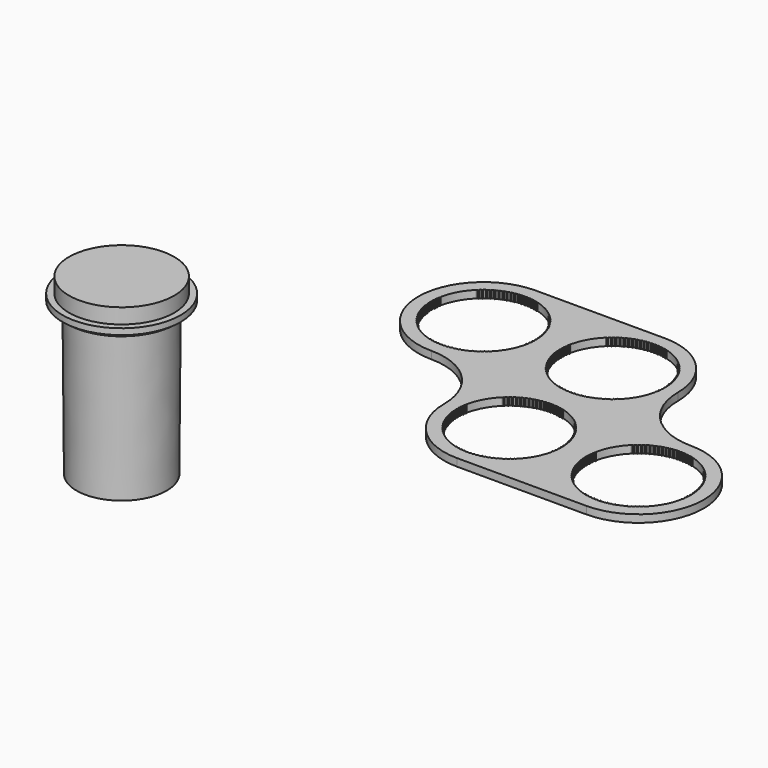
from build123d import *

# Parameters (mm, degrees)
F5_R          = 22.098
F6_DEPTH      = 6.35
F6_DEPTH_BACK = 2.54
F5_R_2        = 24.7948218603
F7_DEPTH      = 2.54
F8_R          = 22.621875
F9_DEPTH      = 1.5875
F10_R         = 19.446875
F12_R         = 18.95078125
F15_DEPTH     = 3.175


# Not quite as in the source:
# - a length typed as a fraction of an inch, garbled in the dataset ("3 / 203.2 mm" for 3/8 in), is restored


with BuildPart() as f6:
    # F5 (on Top) → F6 (new body, two sides)
    with BuildSketch(Plane.XY) as f6_sk:
        Circle(F5_R)
    extrude(amount=F6_DEPTH)
    extrude(f6_sk.sketch, amount=-F6_DEPTH_BACK)

    # F5 (on Top) → F7 (join)
    with BuildSketch(Plane.XY):
        Circle(F5_R_2)
        Circle(F5_R, mode=Mode.SUBTRACT)
    extrude(amount=-F7_DEPTH)


with BuildPart() as f9:
    # F8 (on face) → F9 (new body)
    with BuildSketch(Plane(origin=(0, 0, -2.54), x_dir=(1, 0, 0), z_dir=(0, 0, -1))):
        Circle(F8_R)
    extrude(amount=F9_DEPTH)

    # F10 (on face) → F13 section 0
    with BuildSketch(Plane(origin=(0, 0, -4.1275), x_dir=(1, 0, 0), z_dir=(0, 0, -1))):
        Circle(F10_R)
    # F12 (on offset) → F13 section 1
    with BuildSketch(Plane(origin=(0, 0, -66.83375), x_dir=(1, 0, 0), z_dir=(0, 0, -1))):
        Circle(F12_R)
    loft()


with BuildPart() as f15:
    # F14 (on Top) → F15 (new body)
    with BuildSketch(Plane.XY):
        with BuildLine():
            ThreePointArc((135.5022155802, 0), (143.5290254488, -19.3784332474), (162.9074586963, -27.405243116))
            Line((162.9074586963, -27.405243116), (217.2099449284, -27.405243116))
            ThreePointArc((217.2099449284, -27.405243116), (244.6151880444, 0), (217.2099449284, 27.405243116))
            ThreePointArc((217.2099449284, 27.405243116), (198.1907219258, 35.2832632295), (190.3127018123, 54.3024862321))
            ThreePointArc((190.3127018123, 54.3024862321), (182.2858919437, 73.6809194795), (162.9074586963, 81.7077293481))
            Line((162.9074586963, 81.7077293481), (108.6049724642, 81.7077293481))
            ThreePointArc((108.6049724642, 81.7077293481), (81.1997293481, 54.3024862321), (108.6049724642, 26.897243116))
            ThreePointArc((108.6049724642, 26.897243116), (127.6241954668, 19.0192230026), (135.5022155802, 0))
        make_face()
        with BuildLine():
            Line((184.4449966739, -4.3427294255), (184.3493258728, -4.7928251567))
            ThreePointArc((184.3493258728, -4.7928251567), (182.1607927635, -10.5846099737), (178.4433017857, -15.5358430895))
            Line((178.4433017857, -15.5358430894), (178.1145363694, -15.8577939715))
            Line((178.1145363694, -15.8577939715), (177.6740247135, -15.7247956614))
            Line((177.6740247135, -15.7247956614), (177.7791006262, -16.1727891011))
            Line((177.7791006262, -16.1727891011), (177.4371416893, -16.4806903109))
            Line((177.4371416893, -16.4806903109), (177.0888095533, -16.7813625451))
            Line((177.0888095533, -16.7813625451), (176.6575181795, -16.620966721))
            Line((176.6575181795, -16.620966721), (176.734257008, -17.0746739192))
            Line((176.734257008, -17.0746739192), (176.3736395721, -17.3604957769))
            Line((176.3736395721, -17.3604957769), (176.0071154241, -17.6387027474))
            Line((176.0071154241, -17.6387027474), (175.5867464425, -17.4515424184))
            Line((175.5867464425, -17.4515424184), (175.6348453338, -17.9091728))
            Line((175.6348453338, -17.9091728), (175.2569925911, -18.1717872974))
            Line((175.2569925911, -18.1717872974), (174.8737229346, -18.4264310483))
            Line((174.8737229346, -18.4264310483), (174.4659353494, -18.2132448507))
            Line((174.4659353494, -18.2132448507), (174.4852044791, -18.6729923576))
            Line((174.4852044791, -18.6729923576), (174.0916076417, -18.9113630753))
            Line((174.0916076417, -18.9113630753), (173.6931050669, -19.1414386441))
            Line((173.6931050669, -19.1414386441), (173.2995082295, -18.9030679264))
            Line((173.2995082295, -18.9030679264), (173.2898715512, -19.3631181453))
            Line((173.2898715512, -19.3631181453), (172.882083966, -19.5763043429))
            Line((172.882083966, -19.5763043429), (172.4699211806, -19.7809037265))
            Line((172.4699211806, -19.7809037265), (172.0920684378, -19.518289229))
            Line((172.0920684378, -19.518289229), (172.053563983, -19.9768265519))
            Line((172.053563983, -19.9768265519), (171.6331950014, -20.1639868809))
            Line((171.6331950014, -20.1639868809), (171.2089986235, -20.3423026189))
            Line((171.2089986235, -20.3423026189), (170.8483811875, -20.0564807611))
            Line((170.8483811875, -20.0564807611), (170.7811609157, -20.5116955506))
            Line((170.7811609157, -20.5116955506), (170.349869542, -20.6720913747))
            Line((170.349869542, -20.6720913747), (169.9153136809, -20.8234197363))
            Line((169.9153136809, -20.8234197363), (169.573354744, -20.5155185266))
            Line((169.573354744, -20.5155185266), (169.4776839429, -20.9656142578))
            Line((169.4776839429, -20.9656142578), (169.0371722871, -21.098612568))
            Line((169.0371722871, -21.098612568), (168.5939719362, -21.2223563294))
            Line((168.5939719362, -21.2223563294), (168.2720210541, -20.8935909131))
            Line((168.2720210541, -20.8935909131), (168.1482772927, -21.3367912639))
            Line((168.1482772927, -21.3367912639), (167.700283853, -21.4418671766))
            Line((167.700283853, -21.4418671766), (167.2501881217, -21.5375379776))
            Line((167.2501881217, -21.5375379776), (166.9495158875, -21.1892058416))
            Line((166.9495158875, -21.1892058416), (166.7981875258, -21.6237617027))
            Line((166.7981875258, -21.6237617027), (166.3444803277, -21.7005005312))
            Line((166.3444803277, -21.7005005312), (165.8892655382, -21.767720803))
            Line((165.8892655382, -21.767720803), (165.6110585677, -21.4011966551))
            Line((165.6110585677, -21.4011966551), (165.4327428297, -21.825393033))
            Line((165.4327428297, -21.825393033), (164.9751124482, -21.8734919243))
            Line((164.9751124482, -21.8734919243), (164.5165751254, -21.9119963791))
            Line((164.5165751254, -21.9119963791), (164.2619313744, -21.5287267226))
            Line((164.2619313744, -21.5287267226), (164.0573319909, -21.9408895081))
            Line((164.0573319909, -21.9408895081), (163.597584484, -21.9601586378))
            Line((163.597584484, -21.9601586378), (163.1375342651, -21.9697953161))
            Line((163.1375342651, -21.9697953161), (162.9074586963, -21.5712927414))
            Line((162.9074586963, -21.5712927414), (162.6773831275, -21.9697953161))
            Line((162.6773831275, -21.9697953161), (162.2173329086, -21.9601586378))
            Line((162.2173329086, -21.9601586378), (161.7575854017, -21.9408895081))
            Line((161.7575854017, -21.9408895081), (161.5529860181, -21.5287267226))
            Line((161.5529860181, -21.5287267226), (161.2983422672, -21.9119963791))
            Line((161.2983422672, -21.9119963791), (160.8398049443, -21.8734919243))
            Line((160.8398049443, -21.8734919243), (160.3821745628, -21.825393033))
            Line((160.3821745628, -21.825393033), (160.2038588248, -21.4011966551))
            Line((160.2038588248, -21.4011966551), (159.9256518543, -21.767720803))
            Line((159.9256518543, -21.767720803), (159.4704370649, -21.7005005312))
            Line((159.4704370649, -21.7005005312), (159.0167298667, -21.6237617027))
            Line((159.0167298667, -21.6237617027), (158.8654015051, -21.1892058416))
            Line((158.8654015051, -21.1892058416), (158.5647292708, -21.5375379776))
            Line((158.5647292708, -21.5375379776), (158.1146335395, -21.4418671766))
            Line((158.1146335395, -21.4418671766), (157.6666400998, -21.3367912639))
            Line((157.6666400998, -21.3367912639), (157.5428963384, -20.8935909131))
            Line((157.5428963384, -20.8935909131), (157.2209454563, -21.2223563294))
            Line((157.2209454563, -21.2223563294), (156.7777451055, -21.098612568))
            ThreePointArc((156.7777451055, -21.098612568), (152.3228487226, -19.2533340672), (148.3777757032, -16.4806903108))
            Line((148.3777757032, -16.4806903109), (148.0358167664, -16.1727891011))
            Line((148.0358167664, -16.1727891011), (148.140892679, -15.7247956614))
            Line((148.140892679, -15.7247956614), (147.7003810232, -15.8577939715))
            Line((147.7003810232, -15.8577939715), (147.3716156068, -15.5358430894))
            Line((147.3716156068, -15.5358430894), (147.0496647247, -15.2070776731))
            Line((147.0496647247, -15.2070776731), (147.1826630349, -14.7665660172))
            Line((147.1826630349, -14.7665660172), (146.7346695952, -14.8716419299))
            Line((146.7346695952, -14.8716419299), (146.4267683854, -14.529682993))
            Line((146.4267683854, -14.529682993), (146.1260961511, -14.181350857))
            Line((146.1260961511, -14.181350857), (146.2864919753, -13.7500594832))
            Line((146.2864919753, -13.7500594832), (145.8327847771, -13.8267983118))
            Line((145.8327847771, -13.8267983118), (145.5469629194, -13.4661808758))
            Line((145.5469629194, -13.4661808758), (145.2687559488, -13.0996567279))
            Line((145.2687559488, -13.0996567279), (145.4559162779, -12.6792877463))
            Line((145.4559162779, -12.6792877463), (144.9982858963, -12.7273866375))
            Line((144.9982858963, -12.7273866375), (144.7356713989, -12.3495338948))
            Line((144.7356713989, -12.3495338948), (144.4810276479, -11.9662642383))
            Line((144.4810276479, -11.9662642383), (144.6942138456, -11.5584766532))
            Line((144.6942138456, -11.5584766532), (144.2344663387, -11.5777457829))
            Line((144.2344663387, -11.5777457829), (143.996095621, -11.1841489455))
            Line((143.996095621, -11.1841489455), (143.7660200521, -10.7856463707))
            Line((143.7660200521, -10.7856463707), (144.0043907698, -10.3920495333))
            Line((144.0043907698, -10.3920495333), (143.544340551, -10.3824128549))
            Line((143.544340551, -10.3824128549), (143.3311543533, -9.9746252698))
            Line((143.3311543533, -9.9746252698), (143.1265549698, -9.5624624843))
            Line((143.1265549698, -9.5624624843), (143.3891694672, -9.1846097416))
            Line((143.3891694672, -9.1846097416), (142.9306321444, -9.1461052868))
            Line((142.9306321444, -9.1461052868), (142.7434718154, -8.7257363051))
            Line((142.7434718154, -8.7257363051), (142.5651560774, -8.3015399272))
            Line((142.5651560774, -8.3015399272), (142.8509779351, -7.9409224912))
            Line((142.8509779351, -7.9409224912), (142.3957631457, -7.8737022195))
            Line((142.3957631457, -7.8737022195), (142.2353673216, -7.4424108457))
            Line((142.2353673216, -7.4424108457), (142.0840389599, -7.0078549846))
            Line((142.0840389599, -7.0078549846), (142.3919401697, -6.6658960477))
            Line((142.3919401697, -6.6658960477), (141.9418444384, -6.5702252467))
            Line((141.9418444384, -6.5702252467), (141.8088461283, -6.1297135908))
            Line((141.8088461283, -6.1297135908), (141.6851023669, -5.6865132399))
            Line((141.6851023669, -5.6865132399), (142.0138677832, -5.3645623578))
            Line((142.0138677832, -5.3645623578), (141.5706674324, -5.2408185965))
            Line((141.5706674324, -5.2408185965), (141.4655915197, -4.7928251567))
            Line((141.4655915197, -4.7928251567), (141.3699207187, -4.3427294255))
            Line((141.3699207187, -4.3427294255), (141.7182528547, -4.0420571912))
            Line((141.7182528547, -4.0420571912), (141.2836969936, -3.8907288296))
            Line((141.2836969936, -3.8907288296), (141.2069581651, -3.4370216314))
            Line((141.2069581651, -3.4370216314), (141.1397378933, -2.981806842))
            Line((141.1397378933, -2.981806842), (141.5062620412, -2.7035998714))
            Line((141.5062620412, -2.7035998714), (141.0820656633, -2.5252841335))
            Line((141.0820656633, -2.5252841335), (141.033966772, -2.0676537519))
            Line((141.033966772, -2.0676537519), (140.9954623172, -1.6091164291))
            Line((140.9954623172, -1.6091164291), (141.3787319736, -1.3544726781))
            Line((141.3787319736, -1.3544726781), (140.9665691882, -1.1498732946))
            Line((140.9665691882, -1.1498732946), (140.9473000585, -0.6901257877))
            Line((140.9473000585, -0.6901257877), (140.9376633801, -0.2300755688))
            Line((140.9376633801, -0.2300755688), (141.3361659549, 0))
            Line((141.3361659549, 0), (140.9376633801, 0.2300755688))
            Line((140.9376633801, 0.2300755688), (140.9473000585, 0.6901257877))
            Line((140.9473000585, 0.6901257877), (140.9665691882, 1.1498732946))
            Line((140.9665691882, 1.1498732946), (141.3787319736, 1.3544726781))
            Line((141.3787319736, 1.3544726781), (140.9954623172, 1.6091164291))
            Line((140.9954623172, 1.6091164291), (141.033966772, 2.0676537519))
            Line((141.033966772, 2.0676537519), (141.0820656633, 2.5252841335))
            Line((141.0820656633, 2.5252841335), (141.5062620412, 2.7035998714))
            Line((141.5062620412, 2.7035998714), (141.1397378933, 2.981806842))
            Line((141.1397378933, 2.981806842), (141.2069581651, 3.4370216314))
            Line((141.2069581651, 3.4370216314), (141.2836969936, 3.8907288296))
            Line((141.2836969936, 3.8907288296), (141.7182528547, 4.0420571912))
            Line((141.7182528547, 4.0420571912), (141.3699207187, 4.3427294255))
            Line((141.3699207187, 4.3427294255), (141.4655915197, 4.7928251567))
            ThreePointArc((141.4655915197, 4.7928251567), (143.654124629, 10.5846099737), (147.3716156068, 15.5358430894))
            Line((147.3716156068, 15.5358430894), (147.7003810232, 15.8577939715))
            Line((147.7003810232, 15.8577939715), (148.140892679, 15.7247956614))
            Line((148.140892679, 15.7247956614), (148.0358167664, 16.1727891011))
            Line((148.0358167664, 16.1727891011), (148.3777757032, 16.4806903109))
            Line((148.3777757032, 16.4806903109), (148.7261078393, 16.7813625451))
            Line((148.7261078393, 16.7813625451), (149.157399213, 16.620966721))
            Line((149.157399213, 16.620966721), (149.0806603845, 17.0746739192))
            Line((149.0806603845, 17.0746739192), (149.4412778205, 17.3604957769))
            Line((149.4412778205, 17.3604957769), (149.8078019684, 17.6387027474))
            Line((149.8078019684, 17.6387027474), (150.22817095, 17.4515424184))
            Line((150.22817095, 17.4515424184), (150.1800720587, 17.9091728))
            Line((150.1800720587, 17.9091728), (150.5579248015, 18.1717872974))
            Line((150.5579248015, 18.1717872974), (150.941194458, 18.4264310483))
            Line((150.941194458, 18.4264310483), (151.3489820431, 18.2132448507))
            Line((151.3489820431, 18.2132448507), (151.3297129134, 18.6729923576))
            Line((151.3297129134, 18.6729923576), (151.7233097508, 18.9113630753))
            Line((151.7233097508, 18.9113630753), (152.1218123256, 19.1414386441))
            Line((152.1218123256, 19.1414386441), (152.515409163, 18.9030679264))
            Line((152.515409163, 18.9030679264), (152.5250458413, 19.3631181453))
            Line((152.5250458413, 19.3631181453), (152.9328334265, 19.5763043429))
            Line((152.9328334265, 19.5763043429), (153.344996212, 19.7809037265))
            Line((153.344996212, 19.7809037265), (153.7228489547, 19.518289229))
            Line((153.7228489547, 19.518289229), (153.7613534095, 19.9768265519))
            Line((153.7613534095, 19.9768265519), (154.1817223911, 20.1639868809))
            Line((154.1817223911, 20.1639868809), (154.6059187691, 20.3423026189))
            Line((154.6059187691, 20.3423026189), (154.966536205, 20.0564807611))
            Line((154.966536205, 20.0564807611), (155.0337564768, 20.5116955506))
            Line((155.0337564768, 20.5116955506), (155.4650478506, 20.6720913747))
            Line((155.4650478506, 20.6720913747), (155.8996037117, 20.8234197363))
            Line((155.8996037117, 20.8234197363), (156.2415626486, 20.5155185266))
            Line((156.2415626486, 20.5155185266), (156.3372334496, 20.9656142578))
            Line((156.3372334496, 20.9656142578), (156.7777451055, 21.098612568))
            Line((156.7777451055, 21.098612568), (157.2209454563, 21.2223563294))
            Line((157.2209454563, 21.2223563294), (157.5428963384, 20.8935909131))
            Line((157.5428963384, 20.8935909131), (157.6666400998, 21.3367912639))
            Line((157.6666400998, 21.3367912639), (158.1146335395, 21.4418671766))
            Line((158.1146335395, 21.4418671766), (158.5647292708, 21.5375379776))
            Line((158.5647292708, 21.5375379776), (158.8654015051, 21.1892058416))
            Line((158.8654015051, 21.1892058416), (159.0167298667, 21.6237617027))
            Line((159.0167298667, 21.6237617027), (159.4704370649, 21.7005005312))
            Line((159.4704370649, 21.7005005312), (159.9256518543, 21.767720803))
            Line((159.9256518543, 21.767720803), (160.2038588248, 21.4011966551))
            Line((160.2038588248, 21.4011966551), (160.3821745628, 21.825393033))
            Line((160.3821745628, 21.825393033), (160.8398049443, 21.8734919243))
            Line((160.8398049443, 21.8734919243), (161.2983422672, 21.9119963791))
            Line((161.2983422672, 21.9119963791), (161.5529860181, 21.5287267226))
            Line((161.5529860181, 21.5287267226), (161.7575854017, 21.9408895081))
            Line((161.7575854017, 21.9408895081), (162.2173329086, 21.9601586378))
            Line((162.2173329086, 21.9601586378), (162.6773831275, 21.9697953161))
            Line((162.6773831275, 21.9697953161), (162.9074586963, 21.5712927414))
            Line((162.9074586963, 21.5712927414), (163.1375342651, 21.9697953161))
            Line((163.1375342651, 21.9697953161), (163.597584484, 21.9601586378))
            Line((163.597584484, 21.9601586378), (164.0573319909, 21.9408895081))
            Line((164.0573319909, 21.9408895081), (164.2619313744, 21.5287267226))
            Line((164.2619313744, 21.5287267226), (164.5165751254, 21.9119963791))
            Line((164.5165751254, 21.9119963791), (164.9751124482, 21.8734919243))
            Line((164.9751124482, 21.8734919243), (165.4327428297, 21.825393033))
            Line((165.4327428297, 21.825393033), (165.6110585677, 21.4011966551))
            Line((165.6110585677, 21.4011966551), (165.8892655382, 21.767720803))
            Line((165.8892655382, 21.767720803), (166.3444803277, 21.7005005312))
            Line((166.3444803277, 21.7005005312), (166.7981875258, 21.6237617027))
            Line((166.7981875258, 21.6237617027), (166.9495158875, 21.1892058416))
            Line((166.9495158875, 21.1892058416), (167.2501881217, 21.5375379776))
            Line((167.2501881217, 21.5375379776), (167.700283853, 21.4418671766))
            Line((167.700283853, 21.4418671766), (168.1482772927, 21.3367912639))
            Line((168.1482772927, 21.3367912639), (168.2720210541, 20.8935909131))
            Line((168.2720210541, 20.8935909131), (168.5939719362, 21.2223563294))
            Line((168.5939719362, 21.2223563294), (169.0371722871, 21.098612568))
            ThreePointArc((169.0371722871, 21.098612568), (173.49206867, 19.2533340672), (177.4371416893, 16.4806903109))
            Line((177.4371416893, 16.4806903109), (177.7791006262, 16.1727891011))
            Line((177.7791006262, 16.1727891011), (177.6740247135, 15.7247956614))
            Line((177.6740247135, 15.7247956614), (178.1145363694, 15.8577939715))
            Line((178.1145363694, 15.8577939715), (178.4433017857, 15.5358430894))
            Line((178.4433017857, 15.5358430894), (178.7652526678, 15.2070776731))
            Line((178.7652526678, 15.2070776731), (178.6322543576, 14.7665660172))
            Line((178.6322543576, 14.7665660172), (179.0802477974, 14.8716419299))
            Line((179.0802477974, 14.8716419299), (179.3881490071, 14.529682993))
            Line((179.3881490071, 14.529682993), (179.6888212414, 14.181350857))
            Line((179.6888212414, 14.181350857), (179.5284254173, 13.7500594832))
            Line((179.5284254173, 13.7500594832), (179.9821326154, 13.8267983118))
            Line((179.9821326154, 13.8267983118), (180.2679544732, 13.4661808758))
            Line((180.2679544732, 13.4661808758), (180.5461614437, 13.0996567279))
            Line((180.5461614437, 13.0996567279), (180.3590011147, 12.6792877463))
            Line((180.3590011147, 12.6792877463), (180.8166314962, 12.7273866375))
            Line((180.8166314962, 12.7273866375), (181.0792459937, 12.3495338948))
            Line((181.0792459937, 12.3495338948), (181.3338897446, 11.9662642383))
            Line((181.3338897446, 11.9662642383), (181.120703547, 11.5584766532))
            Line((181.120703547, 11.5584766532), (181.5804510539, 11.5777457829))
            Line((181.5804510539, 11.5777457829), (181.8188217716, 11.1841489455))
            Line((181.8188217716, 11.1841489455), (182.0488973404, 10.7856463707))
            Line((182.0488973404, 10.7856463707), (181.8105266227, 10.3920495333))
            Line((181.8105266227, 10.3920495333), (182.2705768416, 10.3824128549))
            Line((182.2705768416, 10.3824128549), (182.4837630392, 9.9746252698))
            Line((182.4837630392, 9.9746252698), (182.6883624227, 9.5624624843))
            Line((182.6883624227, 9.5624624843), (182.4257479253, 9.1846097416))
            Line((182.4257479253, 9.1846097416), (182.8842852481, 9.1461052868))
            Line((182.8842852481, 9.1461052868), (183.0714455772, 8.7257363051))
            Line((183.0714455772, 8.7257363051), (183.2497613151, 8.3015399272))
            Line((183.2497613151, 8.3015399272), (182.9639394574, 7.9409224912))
            Line((182.9639394574, 7.9409224912), (183.4191542468, 7.8737022195))
            Line((183.4191542468, 7.8737022195), (183.579550071, 7.4424108457))
            Line((183.579550071, 7.4424108457), (183.7308784326, 7.0078549846))
            Line((183.7308784326, 7.0078549846), (183.4229772228, 6.6658960477))
            Line((183.4229772228, 6.6658960477), (183.8730729541, 6.5702252467))
            Line((183.8730729541, 6.5702252467), (184.0060712643, 6.1297135908))
            Line((184.0060712643, 6.1297135908), (184.1298150257, 5.6865132399))
            Line((184.1298150257, 5.6865132399), (183.8010496093, 5.3645623578))
            Line((183.8010496093, 5.3645623578), (184.2442499602, 5.2408185965))
            Line((184.2442499602, 5.2408185965), (184.3493258728, 4.7928251567))
            Line((184.3493258728, 4.7928251567), (184.4449966739, 4.3427294255))
            Line((184.4449966739, 4.3427294255), (184.0966645378, 4.0420571912))
            Line((184.0966645378, 4.0420571912), (184.531220399, 3.8907288296))
            Line((184.531220399, 3.8907288296), (184.6079592275, 3.4370216314))
            Line((184.6079592275, 3.4370216314), (184.6751794993, 2.981806842))
            Line((184.6751794993, 2.981806842), (184.3086553513, 2.7035998714))
            Line((184.3086553513, 2.7035998714), (184.7328517293, 2.5252841335))
            Line((184.7328517293, 2.5252841335), (184.7809506206, 2.0676537519))
            Line((184.7809506206, 2.0676537519), (184.8194550754, 1.6091164291))
            Line((184.8194550754, 1.6091164291), (184.4361854189, 1.3544726781))
            Line((184.4361854189, 1.3544726781), (184.8483482044, 1.1498732946))
            Line((184.8483482044, 1.1498732946), (184.8676173341, 0.6901257877))
            Line((184.8676173341, 0.6901257877), (184.8772540124, 0.2300755688))
            Line((184.8772540124, 0.2300755688), (184.4787514376, 0))
            Line((184.4787514376, 0), (184.8772540124, -0.2300755688))
            Line((184.8772540124, -0.2300755688), (184.8676173341, -0.6901257877))
            Line((184.8676173341, -0.6901257877), (184.8483482044, -1.1498732946))
            Line((184.8483482044, -1.1498732946), (184.4361854189, -1.3544726781))
            Line((184.4361854189, -1.3544726781), (184.8194550754, -1.6091164291))
            Line((184.8194550754, -1.6091164291), (184.7809506206, -2.0676537519))
            Line((184.7809506206, -2.0676537519), (184.7328517293, -2.5252841335))
            Line((184.7328517293, -2.5252841335), (184.3086553513, -2.7035998714))
            Line((184.3086553513, -2.7035998714), (184.6751794993, -2.981806842))
            Line((184.6751794993, -2.981806842), (184.6079592275, -3.4370216314))
            Line((184.6079592275, -3.4370216314), (184.531220399, -3.8907288296))
            Line((184.531220399, -3.8907288296), (184.0966645378, -4.0420571912))
            Line((184.0966645378, -4.0420571912), (184.4449966739, -4.3427294255))
        make_face(mode=Mode.SUBTRACT)
        with BuildLine():
            Line((238.747482906, -4.3427294255), (238.6518121049, -4.7928251567))
            ThreePointArc((238.6518121049, -4.7928251567), (236.4632789956, -10.5846099737), (232.7457880178, -15.5358430895))
            Line((232.7457880178, -15.5358430894), (232.4170226015, -15.8577939715))
            Line((232.4170226015, -15.8577939715), (231.9765109456, -15.7247956614))
            Line((231.9765109456, -15.7247956614), (232.0815868583, -16.1727891011))
            Line((232.0815868583, -16.1727891011), (231.7396279214, -16.4806903109))
            Line((231.7396279214, -16.4806903109), (231.3912957853, -16.7813625451))
            Line((231.3912957853, -16.7813625451), (230.9600044116, -16.620966721))
            Line((230.9600044116, -16.620966721), (231.0367432401, -17.0746739192))
            Line((231.0367432401, -17.0746739192), (230.6761258042, -17.3604957769))
            Line((230.6761258042, -17.3604957769), (230.3096016562, -17.6387027474))
            Line((230.3096016562, -17.6387027474), (229.8892326746, -17.4515424184))
            Line((229.8892326746, -17.4515424184), (229.9373315659, -17.9091728))
            Line((229.9373315659, -17.9091728), (229.5594788231, -18.1717872974))
            Line((229.5594788231, -18.1717872974), (229.1762091667, -18.4264310483))
            Line((229.1762091667, -18.4264310483), (228.7684215815, -18.2132448507))
            Line((228.7684215815, -18.2132448507), (228.7876907112, -18.6729923576))
            Line((228.7876907112, -18.6729923576), (228.3940938738, -18.9113630753))
            Line((228.3940938738, -18.9113630753), (227.995591299, -19.1414386441))
            Line((227.995591299, -19.1414386441), (227.6019944616, -18.9030679264))
            Line((227.6019944616, -18.9030679264), (227.5923577833, -19.3631181453))
            Line((227.5923577833, -19.3631181453), (227.1845701981, -19.5763043429))
            Line((227.1845701981, -19.5763043429), (226.7724074127, -19.7809037265))
            Line((226.7724074127, -19.7809037265), (226.3945546699, -19.518289229))
            Line((226.3945546699, -19.518289229), (226.3560502151, -19.9768265519))
            Line((226.3560502151, -19.9768265519), (225.9356812335, -20.1639868809))
            Line((225.9356812335, -20.1639868809), (225.5114848555, -20.3423026189))
            Line((225.5114848555, -20.3423026189), (225.1508674196, -20.0564807611))
            Line((225.1508674196, -20.0564807611), (225.0836471478, -20.5116955506))
            Line((225.0836471478, -20.5116955506), (224.6523557741, -20.6720913747))
            Line((224.6523557741, -20.6720913747), (224.2177999129, -20.8234197363))
            Line((224.2177999129, -20.8234197363), (223.8758409761, -20.5155185266))
            Line((223.8758409761, -20.5155185266), (223.780170175, -20.9656142578))
            Line((223.780170175, -20.9656142578), (223.3396585191, -21.098612568))
            Line((223.3396585191, -21.098612568), (222.8964581683, -21.2223563294))
            Line((222.8964581683, -21.2223563294), (222.5745072862, -20.8935909131))
            Line((222.5745072862, -20.8935909131), (222.4507635248, -21.3367912639))
            Line((222.4507635248, -21.3367912639), (222.0027700851, -21.4418671766))
            Line((222.0027700851, -21.4418671766), (221.5526743538, -21.5375379776))
            Line((221.5526743538, -21.5375379776), (221.2520021195, -21.1892058416))
            Line((221.2520021195, -21.1892058416), (221.1006737579, -21.6237617027))
            Line((221.1006737579, -21.6237617027), (220.6469665598, -21.7005005312))
            Line((220.6469665598, -21.7005005312), (220.1917517703, -21.767720803))
            Line((220.1917517703, -21.767720803), (219.9135447998, -21.4011966551))
            Line((219.9135447998, -21.4011966551), (219.7352290618, -21.825393033))
            Line((219.7352290618, -21.825393033), (219.2775986803, -21.8734919243))
            Line((219.2775986803, -21.8734919243), (218.8190613575, -21.9119963791))
            Line((218.8190613575, -21.9119963791), (218.5644176065, -21.5287267226))
            Line((218.5644176065, -21.5287267226), (218.359818223, -21.9408895081))
            Line((218.359818223, -21.9408895081), (217.9000707161, -21.9601586378))
            Line((217.9000707161, -21.9601586378), (217.4400204972, -21.9697953161))
            Line((217.4400204972, -21.9697953161), (217.2099449284, -21.5712927414))
            Line((217.2099449284, -21.5712927414), (216.9798693595, -21.9697953161))
            Line((216.9798693595, -21.9697953161), (216.5198191407, -21.9601586378))
            Line((216.5198191407, -21.9601586378), (216.0600716337, -21.9408895081))
            Line((216.0600716337, -21.9408895081), (215.8554722502, -21.5287267226))
            Line((215.8554722502, -21.5287267226), (215.6008284993, -21.9119963791))
            Line((215.6008284993, -21.9119963791), (215.1422911764, -21.8734919243))
            Line((215.1422911764, -21.8734919243), (214.6846607949, -21.825393033))
            Line((214.6846607949, -21.825393033), (214.5063450569, -21.4011966551))
            Line((214.5063450569, -21.4011966551), (214.2281380864, -21.767720803))
            Line((214.2281380864, -21.767720803), (213.772923297, -21.7005005312))
            Line((213.772923297, -21.7005005312), (213.3192160988, -21.6237617027))
            Line((213.3192160988, -21.6237617027), (213.1678877372, -21.1892058416))
            Line((213.1678877372, -21.1892058416), (212.8672155029, -21.5375379776))
            Line((212.8672155029, -21.5375379776), (212.4171197716, -21.4418671766))
            Line((212.4171197716, -21.4418671766), (211.9691263319, -21.3367912639))
            Line((211.9691263319, -21.3367912639), (211.8453825705, -20.8935909131))
            Line((211.8453825705, -20.8935909131), (211.5234316884, -21.2223563294))
            Line((211.5234316884, -21.2223563294), (211.0802313376, -21.098612568))
            ThreePointArc((211.0802313376, -21.098612568), (206.6253349547, -19.2533340672), (202.6802619353, -16.4806903108))
            Line((202.6802619353, -16.4806903109), (202.3383029985, -16.1727891011))
            Line((202.3383029985, -16.1727891011), (202.4433789111, -15.7247956614))
            Line((202.4433789111, -15.7247956614), (202.0028672553, -15.8577939715))
            Line((202.0028672553, -15.8577939715), (201.6741018389, -15.5358430894))
            Line((201.6741018389, -15.5358430894), (201.3521509568, -15.2070776731))
            Line((201.3521509568, -15.2070776731), (201.485149267, -14.7665660172))
            Line((201.485149267, -14.7665660172), (201.0371558273, -14.8716419299))
            Line((201.0371558273, -14.8716419299), (200.7292546175, -14.529682993))
            Line((200.7292546175, -14.529682993), (200.4285823832, -14.181350857))
            Line((200.4285823832, -14.181350857), (200.5889782074, -13.7500594832))
            Line((200.5889782074, -13.7500594832), (200.1352710092, -13.8267983118))
            Line((200.1352710092, -13.8267983118), (199.8494491515, -13.4661808758))
            Line((199.8494491515, -13.4661808758), (199.5712421809, -13.0996567279))
            Line((199.5712421809, -13.0996567279), (199.75840251, -12.6792877463))
            Line((199.75840251, -12.6792877463), (199.3007721284, -12.7273866375))
            Line((199.3007721284, -12.7273866375), (199.038157631, -12.3495338948))
            Line((199.038157631, -12.3495338948), (198.78351388, -11.9662642383))
            Line((198.78351388, -11.9662642383), (198.9967000777, -11.5584766532))
            Line((198.9967000777, -11.5584766532), (198.5369525707, -11.5777457829))
            Line((198.5369525707, -11.5777457829), (198.2985818531, -11.1841489455))
            Line((198.2985818531, -11.1841489455), (198.0685062842, -10.7856463707))
            Line((198.0685062842, -10.7856463707), (198.3068770019, -10.3920495333))
            Line((198.3068770019, -10.3920495333), (197.846826783, -10.3824128549))
            Line((197.846826783, -10.3824128549), (197.6336405854, -9.9746252698))
            Line((197.6336405854, -9.9746252698), (197.4290412019, -9.5624624843))
            Line((197.4290412019, -9.5624624843), (197.6916556993, -9.1846097416))
            Line((197.6916556993, -9.1846097416), (197.2331183765, -9.1461052868))
            Line((197.2331183765, -9.1461052868), (197.0459580475, -8.7257363051))
            Line((197.0459580475, -8.7257363051), (196.8676423095, -8.3015399272))
            Line((196.8676423095, -8.3015399272), (197.1534641672, -7.9409224912))
            Line((197.1534641672, -7.9409224912), (196.6982493778, -7.8737022195))
            Line((196.6982493778, -7.8737022195), (196.5378535537, -7.4424108457))
            Line((196.5378535537, -7.4424108457), (196.386525192, -7.0078549846))
            Line((196.386525192, -7.0078549846), (196.6944264018, -6.6658960477))
            Line((196.6944264018, -6.6658960477), (196.2443306705, -6.5702252467))
            Line((196.2443306705, -6.5702252467), (196.1113323604, -6.1297135908))
            Line((196.1113323604, -6.1297135908), (195.987588599, -5.6865132399))
            Line((195.987588599, -5.6865132399), (196.3163540153, -5.3645623578))
            Line((196.3163540153, -5.3645623578), (195.8731536645, -5.2408185965))
            Line((195.8731536645, -5.2408185965), (195.7680777518, -4.7928251567))
            Line((195.7680777518, -4.7928251567), (195.6724069507, -4.3427294255))
            Line((195.6724069507, -4.3427294255), (196.0207390868, -4.0420571912))
            Line((196.0207390868, -4.0420571912), (195.5861832257, -3.8907288296))
            Line((195.5861832257, -3.8907288296), (195.5094443971, -3.4370216314))
            Line((195.5094443971, -3.4370216314), (195.4422241254, -2.981806842))
            Line((195.4422241254, -2.981806842), (195.8087482733, -2.7035998714))
            Line((195.8087482733, -2.7035998714), (195.3845518954, -2.5252841335))
            Line((195.3845518954, -2.5252841335), (195.3364530041, -2.0676537519))
            Line((195.3364530041, -2.0676537519), (195.2979485493, -1.6091164291))
            Line((195.2979485493, -1.6091164291), (195.6812182057, -1.3544726781))
            Line((195.6812182057, -1.3544726781), (195.2690554203, -1.1498732946))
            Line((195.2690554203, -1.1498732946), (195.2497862906, -0.6901257877))
            Line((195.2497862906, -0.6901257877), (195.2401496122, -0.2300755688))
            Line((195.2401496122, -0.2300755688), (195.638652187, 0))
            Line((195.638652187, 0), (195.2401496122, 0.2300755688))
            Line((195.2401496122, 0.2300755688), (195.2497862906, 0.6901257877))
            Line((195.2497862906, 0.6901257877), (195.2690554203, 1.1498732946))
            Line((195.2690554203, 1.1498732946), (195.6812182057, 1.3544726781))
            Line((195.6812182057, 1.3544726781), (195.2979485493, 1.6091164291))
            Line((195.2979485493, 1.6091164291), (195.3364530041, 2.0676537519))
            Line((195.3364530041, 2.0676537519), (195.3845518954, 2.5252841335))
            Line((195.3845518954, 2.5252841335), (195.8087482733, 2.7035998714))
            Line((195.8087482733, 2.7035998714), (195.4422241254, 2.981806842))
            Line((195.4422241254, 2.981806842), (195.5094443971, 3.4370216314))
            Line((195.5094443971, 3.4370216314), (195.5861832257, 3.8907288296))
            Line((195.5861832257, 3.8907288296), (196.0207390868, 4.0420571912))
            Line((196.0207390868, 4.0420571912), (195.6724069507, 4.3427294255))
            Line((195.6724069507, 4.3427294255), (195.7680777518, 4.7928251567))
            ThreePointArc((195.7680777518, 4.7928251567), (197.9566108611, 10.5846099737), (201.6741018389, 15.5358430895))
            Line((201.6741018389, 15.5358430894), (202.0028672553, 15.8577939715))
            Line((202.0028672553, 15.8577939715), (202.4433789111, 15.7247956614))
            Line((202.4433789111, 15.7247956614), (202.3383029985, 16.1727891011))
            Line((202.3383029985, 16.1727891011), (202.6802619353, 16.4806903109))
            Line((202.6802619353, 16.4806903109), (203.0285940714, 16.7813625451))
            Line((203.0285940714, 16.7813625451), (203.4598854451, 16.620966721))
            Line((203.4598854451, 16.620966721), (203.3831466166, 17.0746739192))
            Line((203.3831466166, 17.0746739192), (203.7437640526, 17.3604957769))
            Line((203.7437640526, 17.3604957769), (204.1102882005, 17.6387027474))
            Line((204.1102882005, 17.6387027474), (204.5306571821, 17.4515424184))
            Line((204.5306571821, 17.4515424184), (204.4825582908, 17.9091728))
            Line((204.4825582908, 17.9091728), (204.8604110336, 18.1717872974))
            Line((204.8604110336, 18.1717872974), (205.24368069, 18.4264310483))
            Line((205.24368069, 18.4264310483), (205.6514682752, 18.2132448507))
            Line((205.6514682752, 18.2132448507), (205.6321991455, 18.6729923576))
            Line((205.6321991455, 18.6729923576), (206.0257959829, 18.9113630753))
            Line((206.0257959829, 18.9113630753), (206.4242985577, 19.1414386441))
            Line((206.4242985577, 19.1414386441), (206.8178953951, 18.9030679264))
            Line((206.8178953951, 18.9030679264), (206.8275320734, 19.3631181453))
            Line((206.8275320734, 19.3631181453), (207.2353196586, 19.5763043429))
            Line((207.2353196586, 19.5763043429), (207.6474824441, 19.7809037265))
            Line((207.6474824441, 19.7809037265), (208.0253351868, 19.518289229))
            Line((208.0253351868, 19.518289229), (208.0638396416, 19.9768265519))
            Line((208.0638396416, 19.9768265519), (208.4842086232, 20.1639868809))
            Line((208.4842086232, 20.1639868809), (208.9084050012, 20.3423026189))
            Line((208.9084050012, 20.3423026189), (209.2690224371, 20.0564807611))
            Line((209.2690224371, 20.0564807611), (209.3362427089, 20.5116955506))
            Line((209.3362427089, 20.5116955506), (209.7675340827, 20.6720913747))
            Line((209.7675340827, 20.6720913747), (210.2020899438, 20.8234197363))
            Line((210.2020899438, 20.8234197363), (210.5440488806, 20.5155185266))
            Line((210.5440488806, 20.5155185266), (210.6397196817, 20.9656142578))
            Line((210.6397196817, 20.9656142578), (211.0802313376, 21.098612568))
            Line((211.0802313376, 21.098612568), (211.5234316884, 21.2223563294))
            Line((211.5234316884, 21.2223563294), (211.8453825705, 20.8935909131))
            Line((211.8453825705, 20.8935909131), (211.9691263319, 21.3367912639))
            Line((211.9691263319, 21.3367912639), (212.4171197716, 21.4418671766))
            Line((212.4171197716, 21.4418671766), (212.8672155029, 21.5375379776))
            Line((212.8672155029, 21.5375379776), (213.1678877372, 21.1892058416))
            Line((213.1678877372, 21.1892058416), (213.3192160988, 21.6237617027))
            Line((213.3192160988, 21.6237617027), (213.772923297, 21.7005005312))
            Line((213.772923297, 21.7005005312), (214.2281380864, 21.767720803))
            Line((214.2281380864, 21.767720803), (214.5063450569, 21.4011966551))
            Line((214.5063450569, 21.4011966551), (214.6846607949, 21.825393033))
            Line((214.6846607949, 21.825393033), (215.1422911764, 21.8734919243))
            Line((215.1422911764, 21.8734919243), (215.6008284993, 21.9119963791))
            Line((215.6008284993, 21.9119963791), (215.8554722502, 21.5287267226))
            Line((215.8554722502, 21.5287267226), (216.0600716337, 21.9408895081))
            Line((216.0600716337, 21.9408895081), (216.5198191407, 21.9601586378))
            Line((216.5198191407, 21.9601586378), (216.9798693595, 21.9697953161))
            Line((216.9798693595, 21.9697953161), (217.2099449284, 21.5712927414))
            Line((217.2099449284, 21.5712927414), (217.4400204972, 21.9697953161))
            Line((217.4400204972, 21.9697953161), (217.9000707161, 21.9601586378))
            Line((217.9000707161, 21.9601586378), (218.359818223, 21.9408895081))
            Line((218.359818223, 21.9408895081), (218.5644176065, 21.5287267226))
            Line((218.5644176065, 21.5287267226), (218.8190613575, 21.9119963791))
            Line((218.8190613575, 21.9119963791), (219.2775986803, 21.8734919243))
            Line((219.2775986803, 21.8734919243), (219.7352290618, 21.825393033))
            Line((219.7352290618, 21.825393033), (219.9135447998, 21.4011966551))
            Line((219.9135447998, 21.4011966551), (220.1917517703, 21.767720803))
            Line((220.1917517703, 21.767720803), (220.6469665598, 21.7005005312))
            Line((220.6469665598, 21.7005005312), (221.1006737579, 21.6237617027))
            Line((221.1006737579, 21.6237617027), (221.2520021195, 21.1892058416))
            Line((221.2520021195, 21.1892058416), (221.5526743538, 21.5375379776))
            Line((221.5526743538, 21.5375379776), (222.0027700851, 21.4418671766))
            Line((222.0027700851, 21.4418671766), (222.4507635248, 21.3367912639))
            Line((222.4507635248, 21.3367912639), (222.5745072862, 20.8935909131))
            Line((222.5745072862, 20.8935909131), (222.8964581683, 21.2223563294))
            Line((222.8964581683, 21.2223563294), (223.3396585191, 21.098612568))
            ThreePointArc((223.3396585191, 21.098612568), (227.794554902, 19.2533340672), (231.7396279214, 16.4806903109))
            Line((231.7396279214, 16.4806903109), (232.0815868583, 16.1727891011))
            Line((232.0815868583, 16.1727891011), (231.9765109456, 15.7247956614))
            Line((231.9765109456, 15.7247956614), (232.4170226015, 15.8577939715))
            Line((232.4170226015, 15.8577939715), (232.7457880178, 15.5358430894))
            Line((232.7457880178, 15.5358430894), (233.0677388999, 15.2070776731))
            Line((233.0677388999, 15.2070776731), (232.9347405897, 14.7665660172))
            Line((232.9347405897, 14.7665660172), (233.3827340295, 14.8716419299))
            Line((233.3827340295, 14.8716419299), (233.6906352392, 14.529682993))
            Line((233.6906352392, 14.529682993), (233.9913074735, 14.181350857))
            Line((233.9913074735, 14.181350857), (233.8309116494, 13.7500594832))
            Line((233.8309116494, 13.7500594832), (234.2846188475, 13.8267983118))
            Line((234.2846188475, 13.8267983118), (234.5704407053, 13.4661808758))
            Line((234.5704407053, 13.4661808758), (234.8486476758, 13.0996567279))
            Line((234.8486476758, 13.0996567279), (234.6614873468, 12.6792877463))
            Line((234.6614873468, 12.6792877463), (235.1191177283, 12.7273866375))
            Line((235.1191177283, 12.7273866375), (235.3817322257, 12.3495338948))
            Line((235.3817322257, 12.3495338948), (235.6363759767, 11.9662642383))
            Line((235.6363759767, 11.9662642383), (235.4231897791, 11.5584766532))
            Line((235.4231897791, 11.5584766532), (235.882937286, 11.5777457829))
            Line((235.882937286, 11.5777457829), (236.1213080037, 11.1841489455))
            Line((236.1213080037, 11.1841489455), (236.3513835725, 10.7856463707))
            Line((236.3513835725, 10.7856463707), (236.1130128548, 10.3920495333))
            Line((236.1130128548, 10.3920495333), (236.5730630737, 10.3824128549))
            Line((236.5730630737, 10.3824128549), (236.7862492713, 9.9746252698))
            Line((236.7862492713, 9.9746252698), (236.9908486548, 9.5624624843))
            Line((236.9908486548, 9.5624624843), (236.7282341574, 9.1846097416))
            Line((236.7282341574, 9.1846097416), (237.1867714802, 9.1461052868))
            Line((237.1867714802, 9.1461052868), (237.3739318093, 8.7257363051))
            Line((237.3739318093, 8.7257363051), (237.5522475472, 8.3015399272))
            Line((237.5522475472, 8.3015399272), (237.2664256895, 7.9409224912))
            Line((237.2664256895, 7.9409224912), (237.7216404789, 7.8737022195))
            Line((237.7216404789, 7.8737022195), (237.8820363031, 7.4424108457))
            Line((237.8820363031, 7.4424108457), (238.0333646647, 7.0078549846))
            Line((238.0333646647, 7.0078549846), (237.7254634549, 6.6658960477))
            Line((237.7254634549, 6.6658960477), (238.1755591862, 6.5702252467))
            Line((238.1755591862, 6.5702252467), (238.3085574964, 6.1297135908))
            Line((238.3085574964, 6.1297135908), (238.4323012578, 5.6865132399))
            Line((238.4323012578, 5.6865132399), (238.1035358414, 5.3645623578))
            Line((238.1035358414, 5.3645623578), (238.5467361923, 5.2408185965))
            Line((238.5467361923, 5.2408185965), (238.6518121049, 4.7928251567))
            Line((238.6518121049, 4.7928251567), (238.747482906, 4.3427294255))
            Line((238.747482906, 4.3427294255), (238.3991507699, 4.0420571912))
            Line((238.3991507699, 4.0420571912), (238.8337066311, 3.8907288296))
            Line((238.8337066311, 3.8907288296), (238.9104454596, 3.4370216314))
            Line((238.9104454596, 3.4370216314), (238.9776657314, 2.981806842))
            Line((238.9776657314, 2.981806842), (238.6111415834, 2.7035998714))
            Line((238.6111415834, 2.7035998714), (239.0353379614, 2.5252841335))
            Line((239.0353379614, 2.5252841335), (239.0834368527, 2.0676537519))
            Line((239.0834368527, 2.0676537519), (239.1219413075, 1.6091164291))
            Line((239.1219413075, 1.6091164291), (238.738671651, 1.3544726781))
            Line((238.738671651, 1.3544726781), (239.1508344365, 1.1498732946))
            Line((239.1508344365, 1.1498732946), (239.1701035662, 0.6901257877))
            Line((239.1701035662, 0.6901257877), (239.1797402445, 0.2300755688))
            Line((239.1797402445, 0.2300755688), (238.7812376697, 0))
            Line((238.7812376697, 0), (239.1797402445, -0.2300755688))
            Line((239.1797402445, -0.2300755688), (239.1701035662, -0.6901257877))
            Line((239.1701035662, -0.6901257877), (239.1508344365, -1.1498732946))
            Line((239.1508344365, -1.1498732946), (238.738671651, -1.3544726781))
            Line((238.738671651, -1.3544726781), (239.1219413075, -1.6091164291))
            Line((239.1219413075, -1.6091164291), (239.0834368527, -2.0676537519))
            Line((239.0834368527, -2.0676537519), (239.0353379614, -2.5252841335))
            Line((239.0353379614, -2.5252841335), (238.6111415834, -2.7035998714))
            Line((238.6111415834, -2.7035998714), (238.9776657314, -2.981806842))
            Line((238.9776657314, -2.981806842), (238.9104454596, -3.4370216314))
            Line((238.9104454596, -3.4370216314), (238.8337066311, -3.8907288296))
            Line((238.8337066311, -3.8907288296), (238.3991507699, -4.0420571912))
            Line((238.3991507699, -4.0420571912), (238.747482906, -4.3427294255))
        make_face(mode=Mode.SUBTRACT)
        with BuildLine():
            Line((130.1425104418, 49.9597568066), (130.0468396407, 49.5096610754))
            ThreePointArc((130.0468396407, 49.5096610754), (127.8583065314, 43.7178762584), (124.1408155536, 38.7666431426))
            Line((124.1408155536, 38.7666431426), (123.8120501373, 38.4446922605))
            Line((123.8120501373, 38.4446922605), (123.3715384814, 38.5776905707))
            Line((123.3715384814, 38.5776905707), (123.4766143941, 38.129697131))
            Line((123.4766143941, 38.129697131), (123.1346554572, 37.8217959212))
            Line((123.1346554572, 37.8217959212), (122.7863233212, 37.521123687))
            Line((122.7863233212, 37.521123687), (122.3550319474, 37.6815195111))
            Line((122.3550319474, 37.6815195111), (122.4317707759, 37.2278123129))
            Line((122.4317707759, 37.2278123129), (122.07115334, 36.9419904552))
            Line((122.07115334, 36.9419904552), (121.704629192, 36.6637834847))
            Line((121.704629192, 36.6637834847), (121.2842602104, 36.8509438137))
            Line((121.2842602104, 36.8509438137), (121.3323591017, 36.3933134321))
            Line((121.3323591017, 36.3933134321), (120.954506359, 36.1306989347))
            Line((120.954506359, 36.1306989347), (120.5712367025, 35.8760551838))
            Line((120.5712367025, 35.8760551838), (120.1634491173, 36.0892413814))
            Line((120.1634491173, 36.0892413814), (120.182718247, 35.6294938745))
            Line((120.182718247, 35.6294938745), (119.7891214096, 35.3911231568))
            Line((119.7891214096, 35.3911231568), (119.3906188349, 35.161047588))
            Line((119.3906188349, 35.161047588), (118.9970219975, 35.3994183057))
            Line((118.9970219975, 35.3994183057), (118.9873853191, 34.9393680868))
            Line((118.9873853191, 34.9393680868), (118.579597734, 34.7261818891))
            Line((118.579597734, 34.7261818891), (118.1674349485, 34.5215825056))
            Line((118.1674349485, 34.5215825056), (117.7895822057, 34.784197003))
            Line((117.7895822057, 34.784197003), (117.7510777509, 34.3256596802))
            Line((117.7510777509, 34.3256596802), (117.3307087693, 34.1384993512))
            Line((117.3307087693, 34.1384993512), (116.9065123914, 33.9601836132))
            Line((116.9065123914, 33.9601836132), (116.5458949554, 34.246005471))
            Line((116.5458949554, 34.246005471), (116.4786746836, 33.7907906815))
            Line((116.4786746836, 33.7907906815), (116.0473833099, 33.6303948574))
            Line((116.0473833099, 33.6303948574), (115.6128274488, 33.4790664958))
            Line((115.6128274488, 33.4790664958), (115.2708685119, 33.7869677055))
            Line((115.2708685119, 33.7869677055), (115.1751977108, 33.3368719743))
            Line((115.1751977108, 33.3368719743), (114.734686055, 33.2038736641))
            Line((114.734686055, 33.2038736641), (114.2914857041, 33.0801299027))
            Line((114.2914857041, 33.0801299027), (113.969534822, 33.408895319))
            Line((113.969534822, 33.408895319), (113.8457910606, 32.9656949682))
            Line((113.8457910606, 32.9656949682), (113.3977976209, 32.8606190555))
            Line((113.3977976209, 32.8606190555), (112.9477018896, 32.7649482545))
            Line((112.9477018896, 32.7649482545), (112.6470296554, 33.1132803905))
            Line((112.6470296554, 33.1132803905), (112.4957012937, 32.6787245294))
            Line((112.4957012937, 32.6787245294), (112.0419940956, 32.6019857009))
            Line((112.0419940956, 32.6019857009), (111.5867793061, 32.5347654291))
            Line((111.5867793061, 32.5347654291), (111.3085723356, 32.901289577))
            Line((111.3085723356, 32.901289577), (111.1302565977, 32.4770931991))
            Line((111.1302565977, 32.4770931991), (110.6726262161, 32.4289943078))
            Line((110.6726262161, 32.4289943078), (110.2140888933, 32.390489853))
            Line((110.2140888933, 32.390489853), (109.9594451423, 32.7737595095))
            Line((109.9594451423, 32.7737595095), (109.7548457588, 32.361596724))
            Line((109.7548457588, 32.361596724), (109.2950982519, 32.3423275943))
            Line((109.2950982519, 32.3423275943), (108.835048033, 32.332690916))
            Line((108.835048033, 32.332690916), (108.6049724642, 32.7311934907))
            Line((108.6049724642, 32.7311934907), (108.3748968954, 32.332690916))
            Line((108.3748968954, 32.332690916), (107.9148466765, 32.3423275943))
            Line((107.9148466765, 32.3423275943), (107.4550991696, 32.361596724))
            Line((107.4550991696, 32.361596724), (107.250499786, 32.7737595095))
            Line((107.250499786, 32.7737595095), (106.9958560351, 32.390489853))
            Line((106.9958560351, 32.390489853), (106.5373187123, 32.4289943078))
            Line((106.5373187123, 32.4289943078), (106.0796883307, 32.4770931991))
            Line((106.0796883307, 32.4770931991), (105.9013725927, 32.901289577))
            Line((105.9013725927, 32.901289577), (105.6231656222, 32.5347654291))
            Line((105.6231656222, 32.5347654291), (105.1679508328, 32.6019857009))
            Line((105.1679508328, 32.6019857009), (104.7142436346, 32.6787245294))
            Line((104.7142436346, 32.6787245294), (104.562915273, 33.1132803905))
            Line((104.562915273, 33.1132803905), (104.2622430387, 32.7649482545))
            Line((104.2622430387, 32.7649482545), (103.8121473075, 32.8606190555))
            Line((103.8121473075, 32.8606190555), (103.3641538677, 32.9656949682))
            Line((103.3641538677, 32.9656949682), (103.2404101063, 33.408895319))
            Line((103.2404101063, 33.408895319), (102.9184592242, 33.0801299027))
            Line((102.9184592242, 33.0801299027), (102.4752588734, 33.2038736641))
            ThreePointArc((102.4752588734, 33.2038736641), (98.0203624905, 35.0491521648), (94.0752894712, 37.8217959212))
            Line((94.0752894712, 37.8217959212), (93.7333305343, 38.129697131))
            Line((93.7333305343, 38.129697131), (93.8384064469, 38.5776905707))
            Line((93.8384064469, 38.5776905707), (93.3978947911, 38.4446922605))
            Line((93.3978947911, 38.4446922605), (93.0691293747, 38.7666431426))
            Line((93.0691293747, 38.7666431426), (92.7471784926, 39.095408559))
            Line((92.7471784926, 39.095408559), (92.8801768028, 39.5359202149))
            Line((92.8801768028, 39.5359202149), (92.4321833631, 39.4308443022))
            Line((92.4321833631, 39.4308443022), (92.1242821533, 39.7728032391))
            Line((92.1242821533, 39.7728032391), (91.823609919, 40.1211353751))
            Line((91.823609919, 40.1211353751), (91.9840057432, 40.5524267489))
            Line((91.9840057432, 40.5524267489), (91.530298545, 40.4756879203))
            Line((91.530298545, 40.4756879203), (91.2444766873, 40.8363053563))
            Line((91.2444766873, 40.8363053563), (90.9662697168, 41.2028295042))
            Line((90.9662697168, 41.2028295042), (91.1534300458, 41.6231984858))
            Line((91.1534300458, 41.6231984858), (90.6957996642, 41.5750995945))
            Line((90.6957996642, 41.5750995945), (90.4331851668, 41.9529523373))
            Line((90.4331851668, 41.9529523373), (90.1785414159, 42.3362219938))
            Line((90.1785414159, 42.3362219938), (90.3917276135, 42.7440095789))
            Line((90.3917276135, 42.7440095789), (89.9319801066, 42.7247404492))
            Line((89.9319801066, 42.7247404492), (89.6936093889, 43.1183372866))
            Line((89.6936093889, 43.1183372866), (89.4635338201, 43.5168398614))
            Line((89.4635338201, 43.5168398614), (89.7019045377, 43.9104366988))
            Line((89.7019045377, 43.9104366988), (89.2418543189, 43.9200733772))
            Line((89.2418543189, 43.9200733772), (89.0286681212, 44.3278609623))
            Line((89.0286681212, 44.3278609623), (88.8240687377, 44.7400237478))
            Line((88.8240687377, 44.7400237478), (89.0866832351, 45.1178764905))
            Line((89.0866832351, 45.1178764905), (88.6281459123, 45.1563809453))
            Line((88.6281459123, 45.1563809453), (88.4409855833, 45.576749927))
            Line((88.4409855833, 45.576749927), (88.2626698453, 46.0009463049))
            Line((88.2626698453, 46.0009463049), (88.5484917031, 46.3615637408))
            Line((88.5484917031, 46.3615637408), (88.0932769136, 46.4287840126))
            Line((88.0932769136, 46.4287840126), (87.9328810895, 46.8600753864))
            Line((87.9328810895, 46.8600753864), (87.7815527279, 47.2946312475))
            Line((87.7815527279, 47.2946312475), (88.0894539376, 47.6365901844))
            Line((88.0894539376, 47.6365901844), (87.6393582063, 47.7322609854))
            Line((87.6393582063, 47.7322609854), (87.5063598962, 48.1727726413))
            Line((87.5063598962, 48.1727726413), (87.3826161348, 48.6159729921))
            Line((87.3826161348, 48.6159729921), (87.7113815511, 48.9379238742))
            Line((87.7113815511, 48.9379238742), (87.2681812003, 49.0616676356))
            Line((87.2681812003, 49.0616676356), (87.1631052876, 49.5096610754))
            Line((87.1631052876, 49.5096610754), (87.0674344866, 49.9597568066))
            Line((87.0674344866, 49.9597568066), (87.4157666226, 50.2604290409))
            Line((87.4157666226, 50.2604290409), (86.9812107615, 50.4117574025))
            Line((86.9812107615, 50.4117574025), (86.904471933, 50.8654646007))
            Line((86.904471933, 50.8654646007), (86.8372516612, 51.3206793901))
            Line((86.8372516612, 51.3206793901), (87.2037758091, 51.5988863607))
            Line((87.2037758091, 51.5988863607), (86.7795794312, 51.7772020986))
            Line((86.7795794312, 51.7772020986), (86.7314805399, 52.2348324802))
            Line((86.7314805399, 52.2348324802), (86.6929760851, 52.693369803))
            Line((86.6929760851, 52.693369803), (87.0762457416, 52.9480135539))
            Line((87.0762457416, 52.9480135539), (86.6640829561, 53.1526129375))
            Line((86.6640829561, 53.1526129375), (86.6448138264, 53.6123604444))
            Line((86.6448138264, 53.6123604444), (86.6351771481, 54.0724106633))
            Line((86.6351771481, 54.0724106633), (87.0336797228, 54.3024862321))
            Line((87.0336797228, 54.3024862321), (86.6351771481, 54.5325618009))
            Line((86.6351771481, 54.5325618009), (86.6448138264, 54.9926120198))
            Line((86.6448138264, 54.9926120198), (86.6640829561, 55.4523595267))
            Line((86.6640829561, 55.4523595267), (87.0762457416, 55.6569589102))
            Line((87.0762457416, 55.6569589102), (86.6929760851, 55.9116026612))
            Line((86.6929760851, 55.9116026612), (86.7314805399, 56.370139984))
            Line((86.7314805399, 56.370139984), (86.7795794312, 56.8277703656))
            Line((86.7795794312, 56.8277703656), (87.2037758091, 57.0060861035))
            Line((87.2037758091, 57.0060861035), (86.8372516612, 57.284293074))
            Line((86.8372516612, 57.284293074), (86.904471933, 57.7395078635))
            Line((86.904471933, 57.7395078635), (86.9812107615, 58.1932150617))
            Line((86.9812107615, 58.1932150617), (87.4157666226, 58.3445434233))
            Line((87.4157666226, 58.3445434233), (87.0674344866, 58.6452156576))
            Line((87.0674344866, 58.6452156576), (87.1631052876, 59.0953113888))
            ThreePointArc((87.1631052876, 59.0953113888), (89.3516383969, 64.8870962058), (93.0691293747, 69.8383293215))
            Line((93.0691293747, 69.8383293215), (93.3978947911, 70.1602802036))
            Line((93.3978947911, 70.1602802036), (93.8384064469, 70.0272818935))
            Line((93.8384064469, 70.0272818935), (93.7333305343, 70.4752753332))
            Line((93.7333305343, 70.4752753332), (94.0752894712, 70.7831765429))
            Line((94.0752894712, 70.7831765429), (94.4236216072, 71.0838487772))
            Line((94.4236216072, 71.0838487772), (94.8549129809, 70.9234529531))
            Line((94.8549129809, 70.9234529531), (94.7781741524, 71.3771601513))
            Line((94.7781741524, 71.3771601513), (95.1387915884, 71.662982009))
            Line((95.1387915884, 71.662982009), (95.5053157363, 71.9411889795))
            Line((95.5053157363, 71.9411889795), (95.9256847179, 71.7540286505))
            Line((95.9256847179, 71.7540286505), (95.8775858266, 72.211659032))
            Line((95.8775858266, 72.211659032), (96.2554385694, 72.4742735295))
            Line((96.2554385694, 72.4742735295), (96.6387082259, 72.7289172804))
            Line((96.6387082259, 72.7289172804), (97.046495811, 72.5157310828))
            Line((97.046495811, 72.5157310828), (97.0272266813, 72.9754785897))
            Line((97.0272266813, 72.9754785897), (97.4208235187, 73.2138493074))
            Line((97.4208235187, 73.2138493074), (97.8193260935, 73.4439248762))
            Line((97.8193260935, 73.4439248762), (98.2129229309, 73.2055541585))
            Line((98.2129229309, 73.2055541585), (98.2225596092, 73.6656043774))
            Line((98.2225596092, 73.6656043774), (98.6303471944, 73.878790575))
            Line((98.6303471944, 73.878790575), (99.0425099799, 74.0833899586))
            Line((99.0425099799, 74.0833899586), (99.4203627226, 73.8207754611))
            Line((99.4203627226, 73.8207754611), (99.4588671774, 74.279312784))
            Line((99.4588671774, 74.279312784), (99.879236159, 74.466473113))
            Line((99.879236159, 74.466473113), (100.303432537, 74.644788851))
            Line((100.303432537, 74.644788851), (100.6640499729, 74.3589669932))
            Line((100.6640499729, 74.3589669932), (100.7312702447, 74.8141817827))
            Line((100.7312702447, 74.8141817827), (101.1625616185, 74.9745776068))
            Line((101.1625616185, 74.9745776068), (101.5971174796, 75.1259059684))
            Line((101.5971174796, 75.1259059684), (101.9390764165, 74.8180047587))
            Line((101.9390764165, 74.8180047587), (102.0347472175, 75.2681004899))
            Line((102.0347472175, 75.2681004899), (102.4752588734, 75.4010988001))
            Line((102.4752588734, 75.4010988001), (102.9184592242, 75.5248425615))
            Line((102.9184592242, 75.5248425615), (103.2404101063, 75.1960771451))
            Line((103.2404101063, 75.1960771451), (103.3641538677, 75.639277496))
            Line((103.3641538677, 75.639277496), (103.8121473075, 75.7443534086))
            Line((103.8121473075, 75.7443534086), (104.2622430387, 75.8400242097))
            Line((104.2622430387, 75.8400242097), (104.562915273, 75.4916920737))
            Line((104.562915273, 75.4916920737), (104.7142436346, 75.9262479348))
            Line((104.7142436346, 75.9262479348), (105.1679508328, 76.0029867633))
            Line((105.1679508328, 76.0029867633), (105.6231656222, 76.0702070351))
            Line((105.6231656222, 76.0702070351), (105.9013725927, 75.7036828871))
            Line((105.9013725927, 75.7036828871), (106.0796883307, 76.1278792651))
            Line((106.0796883307, 76.1278792651), (106.5373187123, 76.1759781564))
            Line((106.5373187123, 76.1759781564), (106.9958560351, 76.2144826112))
            Line((106.9958560351, 76.2144826112), (107.250499786, 75.8312129547))
            Line((107.250499786, 75.8312129547), (107.4550991696, 76.2433757402))
            Line((107.4550991696, 76.2433757402), (107.9148466765, 76.2626448699))
            Line((107.9148466765, 76.2626448699), (108.3748968954, 76.2722815482))
            Line((108.3748968954, 76.2722815482), (108.6049724642, 75.8737789734))
            Line((108.6049724642, 75.8737789734), (108.835048033, 76.2722815482))
            Line((108.835048033, 76.2722815482), (109.2950982519, 76.2626448699))
            Line((109.2950982519, 76.2626448699), (109.7548457588, 76.2433757402))
            Line((109.7548457588, 76.2433757402), (109.9594451423, 75.8312129547))
            Line((109.9594451423, 75.8312129547), (110.2140888933, 76.2144826112))
            Line((110.2140888933, 76.2144826112), (110.6726262161, 76.1759781564))
            Line((110.6726262161, 76.1759781564), (111.1302565977, 76.1278792651))
            Line((111.1302565977, 76.1278792651), (111.3085723356, 75.7036828871))
            Line((111.3085723356, 75.7036828871), (111.5867793061, 76.0702070351))
            Line((111.5867793061, 76.0702070351), (112.0419940956, 76.0029867633))
            Line((112.0419940956, 76.0029867633), (112.4957012937, 75.9262479348))
            Line((112.4957012937, 75.9262479348), (112.6470296554, 75.4916920737))
            Line((112.6470296554, 75.4916920737), (112.9477018896, 75.8400242097))
            Line((112.9477018896, 75.8400242097), (113.3977976209, 75.7443534086))
            Line((113.3977976209, 75.7443534086), (113.8457910606, 75.639277496))
            Line((113.8457910606, 75.639277496), (113.969534822, 75.1960771451))
            Line((113.969534822, 75.1960771451), (114.2914857041, 75.5248425615))
            Line((114.2914857041, 75.5248425615), (114.734686055, 75.4010988001))
            ThreePointArc((114.734686055, 75.4010988001), (119.1895824379, 73.5558202993), (123.1346554572, 70.7831765429))
            Line((123.1346554572, 70.7831765429), (123.4766143941, 70.4752753332))
            Line((123.4766143941, 70.4752753332), (123.3715384814, 70.0272818935))
            Line((123.3715384814, 70.0272818935), (123.8120501373, 70.1602802036))
            Line((123.8120501373, 70.1602802036), (124.1408155536, 69.8383293215))
            Line((124.1408155536, 69.8383293215), (124.4627664357, 69.5095639052))
            Line((124.4627664357, 69.5095639052), (124.3297681256, 69.0690522493))
            Line((124.3297681256, 69.0690522493), (124.7777615653, 69.174128162))
            Line((124.7777615653, 69.174128162), (125.085662775, 68.8321692251))
            Line((125.085662775, 68.8321692251), (125.3863350093, 68.4838370891))
            Line((125.3863350093, 68.4838370891), (125.2259391852, 68.0525457153))
            Line((125.2259391852, 68.0525457153), (125.6796463834, 68.1292845438))
            Line((125.6796463834, 68.1292845438), (125.9654682411, 67.7686671079))
            Line((125.9654682411, 67.7686671079), (126.2436752116, 67.40214296))
            Line((126.2436752116, 67.40214296), (126.0565148826, 66.9817739783))
            Line((126.0565148826, 66.9817739783), (126.5141452641, 67.0298728696))
            Line((126.5141452641, 67.0298728696), (126.7767597616, 66.6520201269))
            Line((126.7767597616, 66.6520201269), (127.0314035125, 66.2687504704))
            Line((127.0314035125, 66.2687504704), (126.8182173149, 65.8609628852))
            Line((126.8182173149, 65.8609628852), (127.2779648218, 65.8802320149))
            Line((127.2779648218, 65.8802320149), (127.5163355395, 65.4866351775))
            Line((127.5163355395, 65.4866351775), (127.7464111083, 65.0881326028))
            Line((127.7464111083, 65.0881326028), (127.5080403906, 64.6945357654))
            Line((127.5080403906, 64.6945357654), (127.9680906095, 64.684899087))
            Line((127.9680906095, 64.684899087), (128.1812768071, 64.2771115019))
            Line((128.1812768071, 64.2771115019), (128.3858761907, 63.8649487164))
            Line((128.3858761907, 63.8649487164), (128.1232616932, 63.4870959736))
            Line((128.1232616932, 63.4870959736), (128.5817990161, 63.4485915188))
            Line((128.5817990161, 63.4485915188), (128.7689593451, 63.0282225372))
            Line((128.7689593451, 63.0282225372), (128.947275083, 62.6040261593))
            Line((128.947275083, 62.6040261593), (128.6614532253, 62.2434087233))
            Line((128.6614532253, 62.2434087233), (129.1166680148, 62.1761884515))
            Line((129.1166680148, 62.1761884515), (129.2770638389, 61.7448970778))
            Line((129.2770638389, 61.7448970778), (129.4283922005, 61.3103412167))
            Line((129.4283922005, 61.3103412167), (129.1204909908, 60.9683822798))
            Line((129.1204909908, 60.9683822798), (129.570586722, 60.8727114787))
            Line((129.570586722, 60.8727114787), (129.7035850322, 60.4321998229))
            Line((129.7035850322, 60.4321998229), (129.8273287936, 59.988999472))
            Line((129.8273287936, 59.988999472), (129.4985633772, 59.6670485899))
            Line((129.4985633772, 59.6670485899), (129.9417637281, 59.5433048285))
            Line((129.9417637281, 59.5433048285), (130.0468396407, 59.0953113888))
            Line((130.0468396407, 59.0953113888), (130.1425104418, 58.6452156576))
            Line((130.1425104418, 58.6452156576), (129.7941783058, 58.3445434233))
            Line((129.7941783058, 58.3445434233), (130.2287341669, 58.1932150617))
            Line((130.2287341669, 58.1932150617), (130.3054729954, 57.7395078635))
            Line((130.3054729954, 57.7395078635), (130.3726932672, 57.284293074))
            Line((130.3726932672, 57.284293074), (130.0061691192, 57.0060861035))
            Line((130.0061691192, 57.0060861035), (130.4303654972, 56.8277703656))
            Line((130.4303654972, 56.8277703656), (130.4784643885, 56.370139984))
            Line((130.4784643885, 56.370139984), (130.5169688433, 55.9116026612))
            Line((130.5169688433, 55.9116026612), (130.1336991868, 55.6569589102))
            Line((130.1336991868, 55.6569589102), (130.5458619723, 55.4523595267))
            Line((130.5458619723, 55.4523595267), (130.565131102, 54.9926120198))
            Line((130.565131102, 54.9926120198), (130.5747677803, 54.5325618009))
            Line((130.5747677803, 54.5325618009), (130.1762652055, 54.3024862321))
            Line((130.1762652055, 54.3024862321), (130.5747677803, 54.0724106633))
            Line((130.5747677803, 54.0724106633), (130.565131102, 53.6123604444))
            Line((130.565131102, 53.6123604444), (130.5458619723, 53.1526129375))
            Line((130.5458619723, 53.1526129375), (130.1336991868, 52.9480135539))
            Line((130.1336991868, 52.9480135539), (130.5169688433, 52.693369803))
            Line((130.5169688433, 52.693369803), (130.4784643885, 52.2348324802))
            Line((130.4784643885, 52.2348324802), (130.4303654972, 51.7772020986))
            Line((130.4303654972, 51.7772020986), (130.0061691192, 51.5988863607))
            Line((130.0061691192, 51.5988863607), (130.3726932672, 51.3206793901))
            Line((130.3726932672, 51.3206793901), (130.3054729954, 50.8654646007))
            Line((130.3054729954, 50.8654646007), (130.2287341669, 50.4117574025))
            Line((130.2287341669, 50.4117574025), (129.7941783058, 50.2604290409))
            Line((129.7941783058, 50.2604290409), (130.1425104418, 49.9597568066))
        make_face(mode=Mode.SUBTRACT)
        with BuildLine():
            Line((184.4449966739, 49.9597568066), (184.3493258728, 49.5096610754))
            ThreePointArc((184.3493258728, 49.5096610754), (182.1607927635, 43.7178762584), (178.4433017857, 38.7666431426))
            Line((178.4433017857, 38.7666431426), (178.1145363694, 38.4446922605))
            Line((178.1145363694, 38.4446922605), (177.6740247135, 38.5776905707))
            Line((177.6740247135, 38.5776905707), (177.7791006262, 38.129697131))
            Line((177.7791006262, 38.129697131), (177.4371416893, 37.8217959212))
            Line((177.4371416893, 37.8217959212), (177.0888095533, 37.521123687))
            Line((177.0888095533, 37.521123687), (176.6575181795, 37.6815195111))
            Line((176.6575181795, 37.6815195111), (176.734257008, 37.2278123129))
            Line((176.734257008, 37.2278123129), (176.3736395721, 36.9419904552))
            Line((176.3736395721, 36.9419904552), (176.0071154241, 36.6637834847))
            Line((176.0071154241, 36.6637834847), (175.5867464425, 36.8509438137))
            Line((175.5867464425, 36.8509438137), (175.6348453338, 36.3933134321))
            Line((175.6348453338, 36.3933134321), (175.2569925911, 36.1306989347))
            Line((175.2569925911, 36.1306989347), (174.8737229346, 35.8760551838))
            Line((174.8737229346, 35.8760551838), (174.4659353494, 36.0892413814))
            Line((174.4659353494, 36.0892413814), (174.4852044791, 35.6294938745))
            Line((174.4852044791, 35.6294938745), (174.0916076417, 35.3911231568))
            Line((174.0916076417, 35.3911231568), (173.6931050669, 35.161047588))
            Line((173.6931050669, 35.161047588), (173.2995082295, 35.3994183057))
            Line((173.2995082295, 35.3994183057), (173.2898715512, 34.9393680868))
            Line((173.2898715512, 34.9393680868), (172.882083966, 34.7261818891))
            Line((172.882083966, 34.7261818891), (172.4699211806, 34.5215825056))
            Line((172.4699211806, 34.5215825056), (172.0920684378, 34.784197003))
            Line((172.0920684378, 34.784197003), (172.053563983, 34.3256596802))
            Line((172.053563983, 34.3256596802), (171.6331950014, 34.1384993512))
            Line((171.6331950014, 34.1384993512), (171.2089986235, 33.9601836132))
            Line((171.2089986235, 33.9601836132), (170.8483811875, 34.246005471))
            Line((170.8483811875, 34.246005471), (170.7811609157, 33.7907906815))
            Line((170.7811609157, 33.7907906815), (170.349869542, 33.6303948574))
            Line((170.349869542, 33.6303948574), (169.9153136809, 33.4790664958))
            Line((169.9153136809, 33.4790664958), (169.573354744, 33.7869677055))
            Line((169.573354744, 33.7869677055), (169.4776839429, 33.3368719743))
            Line((169.4776839429, 33.3368719743), (169.0371722871, 33.2038736641))
            Line((169.0371722871, 33.2038736641), (168.5939719362, 33.0801299027))
            Line((168.5939719362, 33.0801299027), (168.2720210541, 33.408895319))
            Line((168.2720210541, 33.408895319), (168.1482772927, 32.9656949682))
            Line((168.1482772927, 32.9656949682), (167.700283853, 32.8606190555))
            Line((167.700283853, 32.8606190555), (167.2501881217, 32.7649482545))
            Line((167.2501881217, 32.7649482545), (166.9495158875, 33.1132803905))
            Line((166.9495158875, 33.1132803905), (166.7981875258, 32.6787245294))
            Line((166.7981875258, 32.6787245294), (166.3444803277, 32.6019857009))
            Line((166.3444803277, 32.6019857009), (165.8892655382, 32.5347654291))
            Line((165.8892655382, 32.5347654291), (165.6110585677, 32.901289577))
            Line((165.6110585677, 32.901289577), (165.4327428297, 32.4770931991))
            Line((165.4327428297, 32.4770931991), (164.9751124482, 32.4289943078))
            Line((164.9751124482, 32.4289943078), (164.5165751254, 32.390489853))
            Line((164.5165751254, 32.390489853), (164.2619313744, 32.7737595095))
            Line((164.2619313744, 32.7737595095), (164.0573319909, 32.361596724))
            Line((164.0573319909, 32.361596724), (163.597584484, 32.3423275943))
            Line((163.597584484, 32.3423275943), (163.1375342651, 32.332690916))
            Line((163.1375342651, 32.332690916), (162.9074586963, 32.7311934907))
            Line((162.9074586963, 32.7311934907), (162.6773831275, 32.332690916))
            Line((162.6773831275, 32.332690916), (162.2173329086, 32.3423275943))
            Line((162.2173329086, 32.3423275943), (161.7575854017, 32.361596724))
            Line((161.7575854017, 32.361596724), (161.5529860181, 32.7737595095))
            Line((161.5529860181, 32.7737595095), (161.2983422672, 32.390489853))
            Line((161.2983422672, 32.390489853), (160.8398049443, 32.4289943078))
            Line((160.8398049443, 32.4289943078), (160.3821745628, 32.4770931991))
            Line((160.3821745628, 32.4770931991), (160.2038588248, 32.901289577))
            Line((160.2038588248, 32.901289577), (159.9256518543, 32.5347654291))
            Line((159.9256518543, 32.5347654291), (159.4704370649, 32.6019857009))
            Line((159.4704370649, 32.6019857009), (159.0167298667, 32.6787245294))
            Line((159.0167298667, 32.6787245294), (158.8654015051, 33.1132803905))
            Line((158.8654015051, 33.1132803905), (158.5647292708, 32.7649482545))
            Line((158.5647292708, 32.7649482545), (158.1146335395, 32.8606190555))
            Line((158.1146335395, 32.8606190555), (157.6666400998, 32.9656949682))
            Line((157.6666400998, 32.9656949682), (157.5428963384, 33.408895319))
            Line((157.5428963384, 33.408895319), (157.2209454563, 33.0801299027))
            Line((157.2209454563, 33.0801299027), (156.7777451055, 33.2038736641))
            ThreePointArc((156.7777451055, 33.2038736641), (152.3228487226, 35.0491521648), (148.3777757032, 37.8217959212))
            Line((148.3777757032, 37.8217959212), (148.0358167664, 38.129697131))
            Line((148.0358167664, 38.129697131), (148.140892679, 38.5776905707))
            Line((148.140892679, 38.5776905707), (147.7003810232, 38.4446922605))
            Line((147.7003810232, 38.4446922605), (147.3716156068, 38.7666431426))
            Line((147.3716156068, 38.7666431426), (147.0496647247, 39.095408559))
            Line((147.0496647247, 39.095408559), (147.1826630349, 39.5359202149))
            Line((147.1826630349, 39.5359202149), (146.7346695952, 39.4308443022))
            Line((146.7346695952, 39.4308443022), (146.4267683854, 39.7728032391))
            Line((146.4267683854, 39.7728032391), (146.1260961511, 40.1211353751))
            Line((146.1260961511, 40.1211353751), (146.2864919753, 40.5524267489))
            Line((146.2864919753, 40.5524267489), (145.8327847771, 40.4756879203))
            Line((145.8327847771, 40.4756879203), (145.5469629194, 40.8363053563))
            Line((145.5469629194, 40.8363053563), (145.2687559488, 41.2028295042))
            Line((145.2687559488, 41.2028295042), (145.4559162779, 41.6231984858))
            Line((145.4559162779, 41.6231984858), (144.9982858963, 41.5750995945))
            Line((144.9982858963, 41.5750995945), (144.7356713989, 41.9529523373))
            Line((144.7356713989, 41.9529523373), (144.4810276479, 42.3362219938))
            Line((144.4810276479, 42.3362219938), (144.6942138456, 42.7440095789))
            Line((144.6942138456, 42.7440095789), (144.2344663387, 42.7247404492))
            Line((144.2344663387, 42.7247404492), (143.996095621, 43.1183372866))
            Line((143.996095621, 43.1183372866), (143.7660200521, 43.5168398614))
            Line((143.7660200521, 43.5168398614), (144.0043907698, 43.9104366988))
            Line((144.0043907698, 43.9104366988), (143.544340551, 43.9200733772))
            Line((143.544340551, 43.9200733772), (143.3311543533, 44.3278609623))
            Line((143.3311543533, 44.3278609623), (143.1265549698, 44.7400237478))
            Line((143.1265549698, 44.7400237478), (143.3891694672, 45.1178764905))
            Line((143.3891694672, 45.1178764905), (142.9306321444, 45.1563809453))
            Line((142.9306321444, 45.1563809453), (142.7434718154, 45.576749927))
            Line((142.7434718154, 45.576749927), (142.5651560774, 46.0009463049))
            Line((142.5651560774, 46.0009463049), (142.8509779351, 46.3615637408))
            Line((142.8509779351, 46.3615637408), (142.3957631457, 46.4287840126))
            Line((142.3957631457, 46.4287840126), (142.2353673216, 46.8600753864))
            Line((142.2353673216, 46.8600753864), (142.0840389599, 47.2946312475))
            Line((142.0840389599, 47.2946312475), (142.3919401697, 47.6365901844))
            Line((142.3919401697, 47.6365901844), (141.9418444384, 47.7322609854))
            Line((141.9418444384, 47.7322609854), (141.8088461283, 48.1727726413))
            Line((141.8088461283, 48.1727726413), (141.6851023669, 48.6159729921))
            Line((141.6851023669, 48.6159729921), (142.0138677832, 48.9379238742))
            Line((142.0138677832, 48.9379238742), (141.5706674324, 49.0616676356))
            Line((141.5706674324, 49.0616676356), (141.4655915197, 49.5096610754))
            Line((141.4655915197, 49.5096610754), (141.3699207187, 49.9597568066))
            Line((141.3699207187, 49.9597568066), (141.7182528547, 50.2604290409))
            Line((141.7182528547, 50.2604290409), (141.2836969936, 50.4117574025))
            Line((141.2836969936, 50.4117574025), (141.2069581651, 50.8654646007))
            Line((141.2069581651, 50.8654646007), (141.1397378933, 51.3206793901))
            Line((141.1397378933, 51.3206793901), (141.5062620412, 51.5988863607))
            Line((141.5062620412, 51.5988863607), (141.0820656633, 51.7772020986))
            Line((141.0820656633, 51.7772020986), (141.033966772, 52.2348324802))
            Line((141.033966772, 52.2348324802), (140.9954623172, 52.693369803))
            Line((140.9954623172, 52.693369803), (141.3787319736, 52.9480135539))
            Line((141.3787319736, 52.9480135539), (140.9665691882, 53.1526129375))
            Line((140.9665691882, 53.1526129375), (140.9473000585, 53.6123604444))
            Line((140.9473000585, 53.6123604444), (140.9376633801, 54.0724106633))
            Line((140.9376633801, 54.0724106633), (141.3361659549, 54.3024862321))
            Line((141.3361659549, 54.3024862321), (140.9376633801, 54.5325618009))
            Line((140.9376633801, 54.5325618009), (140.9473000585, 54.9926120198))
            Line((140.9473000585, 54.9926120198), (140.9665691882, 55.4523595267))
            Line((140.9665691882, 55.4523595267), (141.3787319736, 55.6569589102))
            Line((141.3787319736, 55.6569589102), (140.9954623172, 55.9116026612))
            Line((140.9954623172, 55.9116026612), (141.033966772, 56.370139984))
            Line((141.033966772, 56.370139984), (141.0820656633, 56.8277703656))
            Line((141.0820656633, 56.8277703656), (141.5062620412, 57.0060861035))
            Line((141.5062620412, 57.0060861035), (141.1397378933, 57.284293074))
            Line((141.1397378933, 57.284293074), (141.2069581651, 57.7395078635))
            Line((141.2069581651, 57.7395078635), (141.2836969936, 58.1932150617))
            Line((141.2836969936, 58.1932150617), (141.7182528547, 58.3445434233))
            Line((141.7182528547, 58.3445434233), (141.3699207187, 58.6452156576))
            Line((141.3699207187, 58.6452156576), (141.4655915197, 59.0953113888))
            ThreePointArc((141.4655915197, 59.0953113888), (143.654124629, 64.8870962058), (147.3716156068, 69.8383293215))
            Line((147.3716156068, 69.8383293215), (147.7003810232, 70.1602802036))
            Line((147.7003810232, 70.1602802036), (148.140892679, 70.0272818935))
            Line((148.140892679, 70.0272818935), (148.0358167664, 70.4752753332))
            Line((148.0358167664, 70.4752753332), (148.3777757032, 70.7831765429))
            Line((148.3777757032, 70.7831765429), (148.7261078393, 71.0838487772))
            Line((148.7261078393, 71.0838487772), (149.157399213, 70.9234529531))
            Line((149.157399213, 70.9234529531), (149.0806603845, 71.3771601513))
            Line((149.0806603845, 71.3771601513), (149.4412778205, 71.662982009))
            Line((149.4412778205, 71.662982009), (149.8078019684, 71.9411889795))
            Line((149.8078019684, 71.9411889795), (150.22817095, 71.7540286505))
            Line((150.22817095, 71.7540286505), (150.1800720587, 72.211659032))
            Line((150.1800720587, 72.211659032), (150.5579248015, 72.4742735295))
            Line((150.5579248015, 72.4742735295), (150.941194458, 72.7289172804))
            Line((150.941194458, 72.7289172804), (151.3489820431, 72.5157310828))
            Line((151.3489820431, 72.5157310828), (151.3297129134, 72.9754785897))
            Line((151.3297129134, 72.9754785897), (151.7233097508, 73.2138493074))
            Line((151.7233097508, 73.2138493074), (152.1218123256, 73.4439248762))
            Line((152.1218123256, 73.4439248762), (152.515409163, 73.2055541585))
            Line((152.515409163, 73.2055541585), (152.5250458413, 73.6656043774))
            Line((152.5250458413, 73.6656043774), (152.9328334265, 73.878790575))
            Line((152.9328334265, 73.878790575), (153.344996212, 74.0833899586))
            Line((153.344996212, 74.0833899586), (153.7228489547, 73.8207754611))
            Line((153.7228489547, 73.8207754611), (153.7613534095, 74.279312784))
            Line((153.7613534095, 74.279312784), (154.1817223911, 74.466473113))
            Line((154.1817223911, 74.466473113), (154.6059187691, 74.644788851))
            Line((154.6059187691, 74.644788851), (154.966536205, 74.3589669932))
            Line((154.966536205, 74.3589669932), (155.0337564768, 74.8141817827))
            Line((155.0337564768, 74.8141817827), (155.4650478506, 74.9745776068))
            Line((155.4650478506, 74.9745776068), (155.8996037117, 75.1259059684))
            Line((155.8996037117, 75.1259059684), (156.2415626486, 74.8180047587))
            Line((156.2415626486, 74.8180047587), (156.3372334496, 75.2681004899))
            Line((156.3372334496, 75.2681004899), (156.7777451055, 75.4010988001))
            Line((156.7777451055, 75.4010988001), (157.2209454563, 75.5248425615))
            Line((157.2209454563, 75.5248425615), (157.5428963384, 75.1960771451))
            Line((157.5428963384, 75.1960771451), (157.6666400998, 75.639277496))
            Line((157.6666400998, 75.639277496), (158.1146335395, 75.7443534086))
            Line((158.1146335395, 75.7443534086), (158.5647292708, 75.8400242097))
            Line((158.5647292708, 75.8400242097), (158.8654015051, 75.4916920737))
            Line((158.8654015051, 75.4916920737), (159.0167298667, 75.9262479348))
            Line((159.0167298667, 75.9262479348), (159.4704370649, 76.0029867633))
            Line((159.4704370649, 76.0029867633), (159.9256518543, 76.0702070351))
            Line((159.9256518543, 76.0702070351), (160.2038588248, 75.7036828871))
            Line((160.2038588248, 75.7036828871), (160.3821745628, 76.1278792651))
            Line((160.3821745628, 76.1278792651), (160.8398049443, 76.1759781564))
            Line((160.8398049443, 76.1759781564), (161.2983422672, 76.2144826112))
            Line((161.2983422672, 76.2144826112), (161.5529860181, 75.8312129547))
            Line((161.5529860181, 75.8312129547), (161.7575854017, 76.2433757402))
            Line((161.7575854017, 76.2433757402), (162.2173329086, 76.2626448699))
            Line((162.2173329086, 76.2626448699), (162.6773831275, 76.2722815482))
            Line((162.6773831275, 76.2722815482), (162.9074586963, 75.8737789734))
            Line((162.9074586963, 75.8737789734), (163.1375342651, 76.2722815482))
            Line((163.1375342651, 76.2722815482), (163.597584484, 76.2626448699))
            Line((163.597584484, 76.2626448699), (164.0573319909, 76.2433757402))
            Line((164.0573319909, 76.2433757402), (164.2619313744, 75.8312129547))
            Line((164.2619313744, 75.8312129547), (164.5165751254, 76.2144826112))
            Line((164.5165751254, 76.2144826112), (164.9751124482, 76.1759781564))
            Line((164.9751124482, 76.1759781564), (165.4327428297, 76.1278792651))
            Line((165.4327428297, 76.1278792651), (165.6110585677, 75.7036828871))
            Line((165.6110585677, 75.7036828871), (165.8892655382, 76.0702070351))
            Line((165.8892655382, 76.0702070351), (166.3444803277, 76.0029867633))
            Line((166.3444803277, 76.0029867633), (166.7981875258, 75.9262479348))
            Line((166.7981875258, 75.9262479348), (166.9495158875, 75.4916920737))
            Line((166.9495158875, 75.4916920737), (167.2501881217, 75.8400242097))
            Line((167.2501881217, 75.8400242097), (167.700283853, 75.7443534086))
            Line((167.700283853, 75.7443534086), (168.1482772927, 75.639277496))
            Line((168.1482772927, 75.639277496), (168.2720210541, 75.1960771451))
            Line((168.2720210541, 75.1960771451), (168.5939719362, 75.5248425615))
            Line((168.5939719362, 75.5248425615), (169.0371722871, 75.4010988001))
            ThreePointArc((169.0371722871, 75.4010988001), (173.49206867, 73.5558202993), (177.4371416893, 70.7831765429))
            Line((177.4371416893, 70.7831765429), (177.7791006262, 70.4752753332))
            Line((177.7791006262, 70.4752753332), (177.6740247135, 70.0272818935))
            Line((177.6740247135, 70.0272818935), (178.1145363694, 70.1602802036))
            Line((178.1145363694, 70.1602802036), (178.4433017857, 69.8383293215))
            Line((178.4433017857, 69.8383293215), (178.7652526678, 69.5095639052))
            Line((178.7652526678, 69.5095639052), (178.6322543576, 69.0690522493))
            Line((178.6322543576, 69.0690522493), (179.0802477974, 69.174128162))
            Line((179.0802477974, 69.174128162), (179.3881490071, 68.8321692251))
            Line((179.3881490071, 68.8321692251), (179.6888212414, 68.4838370891))
            Line((179.6888212414, 68.4838370891), (179.5284254173, 68.0525457153))
            Line((179.5284254173, 68.0525457153), (179.9821326154, 68.1292845438))
            Line((179.9821326154, 68.1292845438), (180.2679544732, 67.7686671079))
            Line((180.2679544732, 67.7686671079), (180.5461614437, 67.40214296))
            Line((180.5461614437, 67.40214296), (180.3590011147, 66.9817739783))
            Line((180.3590011147, 66.9817739783), (180.8166314962, 67.0298728696))
            Line((180.8166314962, 67.0298728696), (181.0792459937, 66.6520201269))
            Line((181.0792459937, 66.6520201269), (181.3338897446, 66.2687504704))
            Line((181.3338897446, 66.2687504704), (181.120703547, 65.8609628852))
            Line((181.120703547, 65.8609628852), (181.5804510539, 65.8802320149))
            Line((181.5804510539, 65.8802320149), (181.8188217716, 65.4866351775))
            Line((181.8188217716, 65.4866351775), (182.0488973404, 65.0881326028))
            Line((182.0488973404, 65.0881326028), (181.8105266227, 64.6945357654))
            Line((181.8105266227, 64.6945357654), (182.2705768416, 64.684899087))
            Line((182.2705768416, 64.684899087), (182.4837630392, 64.2771115019))
            Line((182.4837630392, 64.2771115019), (182.6883624227, 63.8649487164))
            Line((182.6883624227, 63.8649487164), (182.4257479253, 63.4870959736))
            Line((182.4257479253, 63.4870959736), (182.8842852481, 63.4485915188))
            Line((182.8842852481, 63.4485915188), (183.0714455772, 63.0282225372))
            Line((183.0714455772, 63.0282225372), (183.2497613151, 62.6040261593))
            Line((183.2497613151, 62.6040261593), (182.9639394574, 62.2434087233))
            Line((182.9639394574, 62.2434087233), (183.4191542468, 62.1761884515))
            Line((183.4191542468, 62.1761884515), (183.579550071, 61.7448970778))
            Line((183.579550071, 61.7448970778), (183.7308784326, 61.3103412167))
            Line((183.7308784326, 61.3103412167), (183.4229772228, 60.9683822798))
            Line((183.4229772228, 60.9683822798), (183.8730729541, 60.8727114787))
            Line((183.8730729541, 60.8727114787), (184.0060712643, 60.4321998229))
            Line((184.0060712643, 60.4321998229), (184.1298150257, 59.988999472))
            Line((184.1298150257, 59.988999472), (183.8010496093, 59.6670485899))
            Line((183.8010496093, 59.6670485899), (184.2442499602, 59.5433048285))
            Line((184.2442499602, 59.5433048285), (184.3493258728, 59.0953113888))
            Line((184.3493258728, 59.0953113888), (184.4449966739, 58.6452156576))
            Line((184.4449966739, 58.6452156576), (184.0966645378, 58.3445434233))
            Line((184.0966645378, 58.3445434233), (184.531220399, 58.1932150617))
            Line((184.531220399, 58.1932150617), (184.6079592275, 57.7395078635))
            Line((184.6079592275, 57.7395078635), (184.6751794993, 57.284293074))
            Line((184.6751794993, 57.284293074), (184.3086553513, 57.0060861035))
            Line((184.3086553513, 57.0060861035), (184.7328517293, 56.8277703656))
            Line((184.7328517293, 56.8277703656), (184.7809506206, 56.370139984))
            Line((184.7809506206, 56.370139984), (184.8194550754, 55.9116026612))
            Line((184.8194550754, 55.9116026612), (184.4361854189, 55.6569589102))
            Line((184.4361854189, 55.6569589102), (184.8483482044, 55.4523595267))
            Line((184.8483482044, 55.4523595267), (184.8676173341, 54.9926120198))
            Line((184.8676173341, 54.9926120198), (184.8772540124, 54.5325618009))
            Line((184.8772540124, 54.5325618009), (184.4787514376, 54.3024862321))
            Line((184.4787514376, 54.3024862321), (184.8772540124, 54.0724106633))
            Line((184.8772540124, 54.0724106633), (184.8676173341, 53.6123604444))
            Line((184.8676173341, 53.6123604444), (184.8483482044, 53.1526129375))
            Line((184.8483482044, 53.1526129375), (184.4361854189, 52.9480135539))
            Line((184.4361854189, 52.9480135539), (184.8194550754, 52.693369803))
            Line((184.8194550754, 52.693369803), (184.7809506206, 52.2348324802))
            Line((184.7809506206, 52.2348324802), (184.7328517293, 51.7772020986))
            Line((184.7328517293, 51.7772020986), (184.3086553513, 51.5988863607))
            Line((184.3086553513, 51.5988863607), (184.6751794993, 51.3206793901))
            Line((184.6751794993, 51.3206793901), (184.6079592275, 50.8654646007))
            Line((184.6079592275, 50.8654646007), (184.531220399, 50.4117574025))
            Line((184.531220399, 50.4117574025), (184.0966645378, 50.2604290409))
            Line((184.0966645378, 50.2604290409), (184.4449966739, 49.9597568066))
        make_face(mode=Mode.SUBTRACT)
    extrude(amount=F15_DEPTH)


solid = Compound([f6.part, f9.part, f15.part])
